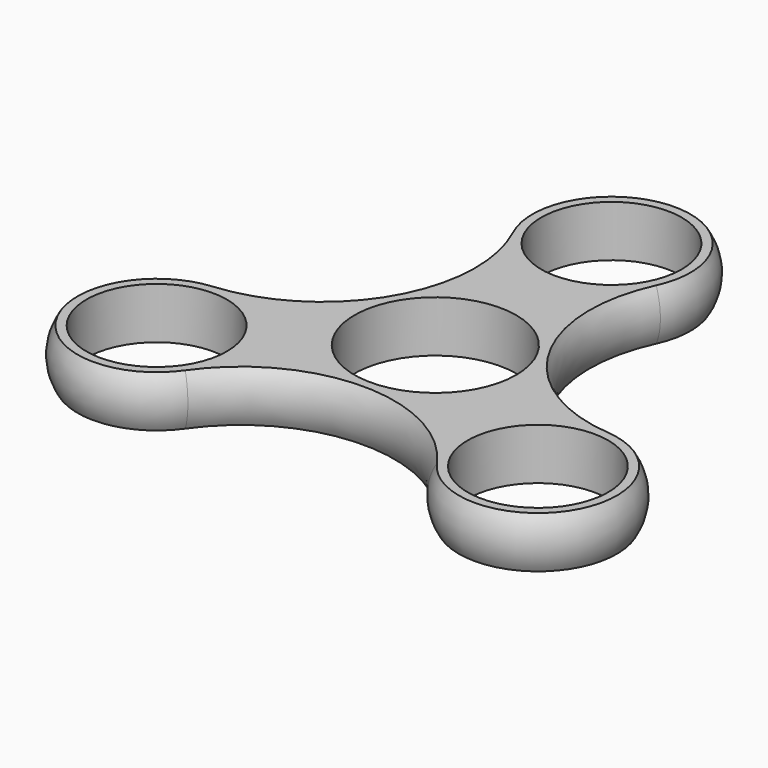
from build123d import *

# Parameters (mm, degrees)
F0_R     = 9.575
F0_R_2   = 11.025
F1_DEPTH = 3.5


# Not quite as in the source:
# - a feature names something its author has since deleted; it is built from what else it names


with BuildPart() as f1:
    # F0 (on Top) → F1 (new body, symmetric)
    with BuildSketch(Plane.XY):
        with BuildLine():
            ThreePointArc((-9.7584878157, 25.4313524375), (-10.5871605613, 6.1125), (-26.9034411714, -4.2645778678))
            ThreePointArc((-26.9034411714, -4.2645778678), (-35.3121858393, -20.3875), (-17.1449533556, -21.1667745697))
            ThreePointArc((-17.1449533556, -21.1667745697), (0, -12.225), (17.1449533556, -21.1667745697))
            ThreePointArc((17.1449533556, -21.1667745697), (35.3121858393, -20.3875), (26.9034411714, -4.2645778678))
            ThreePointArc((26.9034411714, -4.2645778678), (10.5871605613, 6.1125), (9.7584878157, 25.4313524375))
            ThreePointArc((9.7584878157, 25.4313524375), (0, 40.775), (-9.7584878157, 25.4313524375))
        make_face()
        with Locations((-25.9807621135, -15)):
            Circle(F0_R, mode=Mode.SUBTRACT)
        Circle(F0_R_2, mode=Mode.SUBTRACT)
        with Locations((25.9807621135, -15)):
            Circle(F0_R, mode=Mode.SUBTRACT)
        with Locations((0, 30)):
            Circle(F0_R, mode=Mode.SUBTRACT)
    extrude(amount=F1_DEPTH, both=True)

    # F4: sweep along a path in F0
    with BuildLine(Plane.XY) as f4_path:
        ThreePointArc((9.7584878157, 25.4313524375), (0, 40.775), (-9.7584878157, 25.4313524375))
    # F3 (on line) → F4 (sweep)
    with BuildSketch(Plane(origin=(11.5201166848, 24.6066077034, 0), x_dir=(-0.9056601221, 0.4240044141, 0), z_dir=(0.4240044141, 0.9056601221, 0))):
        with BuildLine():
            ThreePointArc((1.9451324245, 3.5), (0.9451324245, 0), (1.9451324245, -3.5))
            Line((1.9451324245, -3.5), (1.9451324245, 3.5))
        make_face()
    sweep(path=f4_path.line)

    # F5: sweep along a path in F0
    with BuildLine(Plane.XY) as f5_path:
        ThreePointArc((9.7584878157, 25.4313524375), (10.5871605613, 6.1125), (26.9034411714, -4.2645778678))
        ThreePointArc((26.9034411714, -4.2645778678), (35.3121858393, -20.3875), (17.1449533556, -21.1667745697))
        ThreePointArc((17.1449533556, -21.1667745697), (0, -12.225), (-17.1449533556, -21.1667745697))
        ThreePointArc((-17.1449533556, -21.1667745697), (-35.3121858393, -20.3875), (-26.9034411714, -4.2645778678))
        ThreePointArc((-26.9034411714, -4.2645778678), (-10.5871605613, 6.1125), (-9.7584878157, 25.4313524375))
    # F4_face (on face) → F5 (sweep)
    with BuildSketch(Plane(origin=(10.1232025909, 25.2606033113, 0), x_dir=(0.9056601221, -0.4240044141, 0), z_dir=(-0.4240044141, -0.9056601221, 0))):
        with BuildLine():
            ThreePointArc((-0.402706011, -3.5), (0.597293989, 0), (-0.402706011, 3.5))
            Line((-0.402706011, 3.5), (-0.402706011, -3.5))
        make_face()
    sweep(path=f5_path.line)


solid = f1.part
